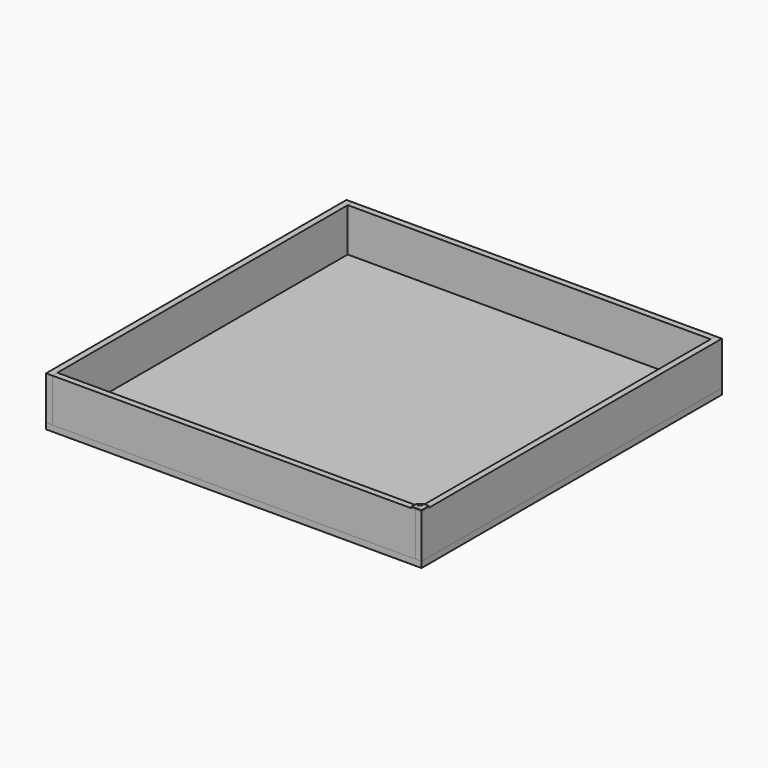
from build123d import *

# Parameters (mm, degrees)
F0_W      = 1207
F0_H      = 1207
F1_DEPTH  = 19.05
F2_W      = 20.2
F2_H      = 1207
F3_DEPTH  = 139.7
F5_W      = 1166.6
F5_H      = 20.2
F6_DEPTH  = 139.7
F10_DEPTH = 5
F12_DEPTH = 8
F14_DEPTH = 5
F15_R     = 1


# Not quite as in the source:
# - two fillets or chamfers of one size are made in one step


with BuildPart() as f1:
    # F0 (on Top) → F1 (new body)
    with BuildSketch(Plane.XY):
        Rectangle(F0_W, F0_H)
    extrude(amount=F1_DEPTH)


with BuildPart() as f3:
    # F2 (on face) → F3 (new body)
    with BuildSketch(Plane.XY.offset(19.05)):
        with Locations((-593.4, 0)):
            Rectangle(F2_W, F2_H)
    extrude(amount=F3_DEPTH)


with BuildPart() as f4_1:
    # F4: instance of F3
    add(f3.part.mirror(Plane.YZ))


with BuildPart() as f6:
    # F5 (on face) → F6 (new body)
    with BuildSketch(Plane.XY.offset(19.05)):
        with Locations((0, 593.4)):
            Rectangle(F5_W, F5_H)
    extrude(amount=F6_DEPTH)


with BuildPart() as f7_1:
    # F7: instance of F6
    add(f6.part.mirror(Plane.XZ))


with BuildPart() as f10:
    # F9 (on offset) → F10 (new body)
    with BuildSketch(Plane.XY.offset(158.75)):
        Polygon((585.4039892925, -572.7107293333), (583.3, -574.8147186258), (583.3, -580.4715728753), (586.9769552622, -576.7946176131), (588.3911688245, -578.2088311755), (589.8053823869, -579.6230447378), (583.3, -586.1284271247), (583.3, -591.7852813742), (593.8063995238, -581.2788818505), align=None)
        Polygon((583.3, -580.4715728753), (583.3, -574.8147186258), (574.8147186258, -583.3), (580.4715728753, -583.3), align=None)
        Polygon((580.4715728753, -583.3), (574.8147186258, -583.3), (571.1377633636, -586.9769552622), (579.6230447378, -595.4622366364), (583.3, -591.7852813742), (583.3, -586.1284271247), (579.6230447378, -589.8053823869), (578.2088311755, -588.3911688245), (576.7946176131, -586.9769552622), align=None)
    extrude(amount=F10_DEPTH)

    # F11 (on face) → F12 (join)
    with BuildSketch(Plane(origin=(0, 0, 158.75), x_dir=(1, 0, 0), z_dir=(0, 0, -1))):
        Polygon((583.3, 583.3), (574.8147186258, 583.3), (583.3, 574.8147186258), align=None)
    extrude(amount=F12_DEPTH)

    # F13 (on face) → F14 (join)
    with BuildSketch(Plane.XY.offset(158.75)):
        Polygon((603.5, -572.7107293333), (585.4039892925, -572.7107293333), (571.1377633636, -586.9769552622), (571.1377633636, -603.5), (583.3, -603.5), (603.5, -603.5), align=None)
        Polygon((576.7946176131, -586.9769552622), (586.9769552622, -576.7946176131), (589.8053823869, -579.6230447378), (579.6230447378, -589.8053823869), align=None, mode=Mode.SUBTRACT)
    extrude(amount=F14_DEPTH)

    # F15
    f15_edges = [f10.edges().sort_by_distance(p)[0] for p in [
        (578.270876, -579.843842, 163.75),
        (571.137763, -603.5, 161.25),
        (571.137763, -595.238478, 163.75),
        (587.318882, -603.5, 163.75),
        (603.5, -588.105365, 163.75),
        (594.451995, -572.710729, 163.75),
        (603.5, -572.710729, 161.25),
    ]]
    fillet(f15_edges, radius=F15_R)


solid = Compound([f1.part, f3.part, f4_1.part, f6.part, f7_1.part, f10.part])
